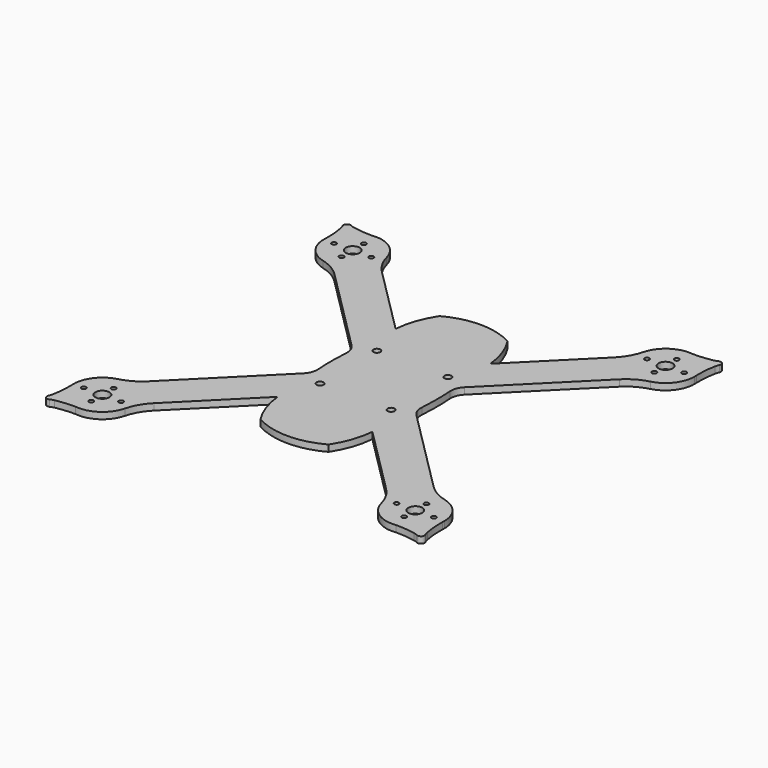
from build123d import *

# Parameters (mm, degrees)
F0_R     = 1
F0_R_2   = 3
F0_R_3   = 1.5
F1_DEPTH = 2.8


# Not quite as in the source:
# - a feature names something its author has since deleted; it is built from what else it names


with BuildPart() as f1:
    # F0 (on Top) → F1 (new body)
    with BuildSketch(Plane.XY):
        with BuildLine():
            ThreePointArc((-24.2769210382, 12.9632125392), (-22.6715914724, 10.4692673994), (-22.2430782145, 7.5344383136))
            add(Edge.make_bspline(
                [(-22.2430782145, 7.5344383136), (-22.7598893965, 0), (-22.2430782145, -7.5344383136)],
                knots=[1.419531369, 1.419531369, 1.419531369, 1.7220612846, 1.7220612846, 1.7220612846], degree=2, weights=[1, 0.988581254, 1]))
            ThreePointArc((-22.2430782145, -7.5344383136), (-22.6715914724, -10.4692673994), (-24.2769210382, -12.9632125392))
            Line((-24.2769210382, -12.9632125392), (-61.1647365726, -49.8510280737))
            ThreePointArc((-61.1647365726, -49.8510280737), (-65.3840934292, -53.0737552924), (-70.3027318987, -55.0727396886))
            ThreePointArc((-70.3027318987, -55.0727396886), (-77.058080165, -59.5215452578), (-79.6751442127, -67.1751442127))
            ThreePointArc((-79.6751442127, -67.1751442127), (-79.6503390116, -67.6938343507), (-79.6320011275, -68.2127933849))
            ThreePointArc((-79.6320011275, -68.2127933849), (-79.7454623748, -72.7266284611), (-80.3467756366, -77.2016706856))
            ThreePointArc((-80.3467756366, -77.2016706856), (-80.5705641186, -78.0710076077), (-80.9037667053, -78.9045566495))
            ThreePointArc((-80.9037667053, -78.9045566495), (-80.607151465, -80.6131466395), (-78.8969122154, -80.9000997088))
            ThreePointArc((-78.8969122154, -80.9000997088), (-78.065259844, -80.5621909904), (-77.1972017245, -80.3334923456))
            ThreePointArc((-77.1972017245, -80.3334923456), (-73.0608106601, -79.7368187673), (-68.8854512989, -79.5575853965))
            ThreePointArc((-68.8854512989, -79.5575853965), (-60.2172709309, -77.5596518753), (-55.0727396886, -70.3027318987))
            ThreePointArc((-55.0727396886, -70.3027318987), (-53.0737552924, -65.3840934292), (-49.8510280737, -61.1647365726))
            Line((-49.8510280737, -61.1647365726), (-20.3225413072, -31.6362498062))
            ThreePointArc((-20.3225413072, -31.6362498062), (-18.4728822052, -40.1836633503), (-14.6194240078, -48.0341650546))
            ThreePointArc((-14.6194240078, -48.0341650546), (0, -51.7838309168), (14.6194240078, -48.0341650546))
            ThreePointArc((14.6194240078, -48.0341650546), (18.4728822052, -40.1836633503), (20.3225413072, -31.6362498062))
            Line((20.3225413072, -31.6362498062), (49.8510280737, -61.1647365726))
            ThreePointArc((49.8510280737, -61.1647365726), (53.0737552924, -65.3840934292), (55.0727396886, -70.3027318987))
            ThreePointArc((55.0727396886, -70.3027318987), (60.2172709309, -77.5596518753), (68.8854512989, -79.5575853965))
            ThreePointArc((68.8854512989, -79.5575853965), (73.0608106601, -79.7368187673), (77.1972017245, -80.3334923456))
            ThreePointArc((77.1972017245, -80.3334923456), (78.065259844, -80.5621909904), (78.8969122154, -80.9000997088))
            ThreePointArc((78.8969122154, -80.9000997088), (80.607151465, -80.6131466395), (80.9037667053, -78.9045566495))
            ThreePointArc((80.9037667053, -78.9045566495), (80.5705641186, -78.0710076077), (80.3467756366, -77.2016706856))
            ThreePointArc((80.3467756366, -77.2016706856), (79.7454623748, -72.7266284611), (79.6320011275, -68.2127933849))
            ThreePointArc((79.6320011275, -68.2127933849), (79.6503390116, -67.6938343507), (79.6751442127, -67.1751442127))
            ThreePointArc((79.6751442127, -67.1751442127), (77.058080165, -59.5215452578), (70.3027318987, -55.0727396886))
            ThreePointArc((70.3027318987, -55.0727396886), (65.3840934292, -53.0737552924), (61.1647365726, -49.8510280737))
            Line((61.1647365726, -49.8510280737), (24.2769210382, -12.9632125392))
            ThreePointArc((24.2769210382, -12.9632125392), (22.6715914724, -10.4692673994), (22.2430782145, -7.5344383136))
            add(Edge.make_bspline(
                [(22.2430782145, -7.5344383136), (22.7598893965, 0), (22.2430782145, 7.5344383136)],
                knots=[4.5611240226, 4.5611240226, 4.5611240226, 4.8636539382, 4.8636539382, 4.8636539382], degree=2, weights=[1, 0.988581254, 1]))
            ThreePointArc((22.2430782145, 7.5344383136), (22.6715914724, 10.4692673994), (24.2769210382, 12.9632125392))
            Line((24.2769210382, 12.9632125392), (61.1647365726, 49.8510280737))
            ThreePointArc((61.1647365726, 49.8510280737), (65.3840934292, 53.0737552924), (70.3027318987, 55.0727396886))
            ThreePointArc((70.3027318987, 55.0727396886), (77.058080165, 59.5215452578), (79.6751442127, 67.1751442127))
            ThreePointArc((79.6751442127, 67.1751442127), (79.6503390116, 67.6938343507), (79.6320011275, 68.2127933849))
            ThreePointArc((79.6320011275, 68.2127933849), (79.7454623748, 72.7266284611), (80.3467756366, 77.2016706856))
            ThreePointArc((80.3467756366, 77.2016706856), (80.5705641186, 78.0710076077), (80.9037667053, 78.9045566495))
            ThreePointArc((80.9037667053, 78.9045566495), (80.607151465, 80.6131466395), (78.8969122154, 80.9000997088))
            ThreePointArc((78.8969122154, 80.9000997088), (78.065259844, 80.5621909904), (77.1972017245, 80.3334923456))
            ThreePointArc((77.1972017245, 80.3334923456), (73.0608106601, 79.7368187673), (68.8854512989, 79.5575853965))
            ThreePointArc((68.8854512989, 79.5575853965), (60.2172709309, 77.5596518753), (55.0727396886, 70.3027318987))
            ThreePointArc((55.0727396886, 70.3027318987), (53.0737552924, 65.3840934292), (49.8510280737, 61.1647365726))
            Line((49.8510280737, 61.1647365726), (20.3225413072, 31.6362498062))
            ThreePointArc((20.3225413072, 31.6362498062), (18.4728822052, 40.1836633503), (14.6194240078, 48.0341650546))
            ThreePointArc((14.6194240078, 48.0341650546), (0, 51.7838309168), (-14.6194240078, 48.0341650546))
            ThreePointArc((-14.6194240078, 48.0341650546), (-18.4728822052, 40.1836633503), (-20.3225413072, 31.6362498062))
            Line((-20.3225413072, 31.6362498062), (-49.8510280737, 61.1647365726))
            ThreePointArc((-49.8510280737, 61.1647365726), (-53.0737552924, 65.3840934292), (-55.0727396886, 70.3027318987))
            ThreePointArc((-55.0727396886, 70.3027318987), (-60.2172709309, 77.5596518753), (-68.8854512989, 79.5575853965))
            ThreePointArc((-68.8854512989, 79.5575853965), (-73.0608106601, 79.7368187673), (-77.1972017245, 80.3334923456))
            ThreePointArc((-77.1972017245, 80.3334923456), (-78.065259844, 80.5621909904), (-78.8969122154, 80.9000997088))
            ThreePointArc((-78.8969122154, 80.9000997088), (-80.607151465, 80.6131466395), (-80.9037667053, 78.9045566495))
            ThreePointArc((-80.9037667053, 78.9045566495), (-80.5705641186, 78.0710076077), (-80.3467756366, 77.2016706856))
            ThreePointArc((-80.3467756366, 77.2016706856), (-79.7454623748, 72.7266284611), (-79.6320011275, 68.2127933849))
            ThreePointArc((-79.6320011275, 68.2127933849), (-79.6503390116, 67.6938343507), (-79.6751442127, 67.1751442127))
            ThreePointArc((-79.6751442127, 67.1751442127), (-77.058080165, 59.5215452578), (-70.3027318987, 55.0727396886))
            ThreePointArc((-70.3027318987, 55.0727396886), (-65.3840934292, 53.0737552924), (-61.1647365726, 49.8510280737))
            Line((-61.1647365726, 49.8510280737), (-24.2769210382, 12.9632125392))
        make_face()
        with Locations((-67.1751442127, -73.1751442127)):
            Circle(F0_R, mode=Mode.SUBTRACT)
        with Locations((-75.1751442127, -67.1751442127)):
            Circle(F0_R, mode=Mode.SUBTRACT)
        with Locations((-67.1751442127, -67.1751442127)):
            Circle(F0_R_2, mode=Mode.SUBTRACT)
        with Locations((-67.1751442127, -61.1751442127)):
            Circle(F0_R, mode=Mode.SUBTRACT)
        with Locations((-59.1751442127, -67.1751442127)):
            Circle(F0_R, mode=Mode.SUBTRACT)
        with Locations((-15.25, -15.25)):
            Circle(F0_R_3, mode=Mode.SUBTRACT)
        with Locations((59.1751442127, -67.1751442127)):
            Circle(F0_R, mode=Mode.SUBTRACT)
        with Locations((67.1751442127, -73.1751442127)):
            Circle(F0_R, mode=Mode.SUBTRACT)
        with Locations((67.1751442127, -67.1751442127)):
            Circle(F0_R_2, mode=Mode.SUBTRACT)
        with Locations((67.1751442127, -61.1751442127)):
            Circle(F0_R, mode=Mode.SUBTRACT)
        with Locations((75.1751442127, -67.1751442127)):
            Circle(F0_R, mode=Mode.SUBTRACT)
        with Locations((15.25, -15.25)):
            Circle(F0_R_3, mode=Mode.SUBTRACT)
        with Locations((-15.25, 15.25)):
            Circle(F0_R_3, mode=Mode.SUBTRACT)
        with Locations((-75.1751442127, 67.1751442127)):
            Circle(F0_R, mode=Mode.SUBTRACT)
        with Locations((-67.1751442127, 61.1751442127)):
            Circle(F0_R, mode=Mode.SUBTRACT)
        with Locations((-67.1751442127, 67.1751442127)):
            Circle(F0_R_2, mode=Mode.SUBTRACT)
        with Locations((-67.1751442127, 73.1751442127)):
            Circle(F0_R, mode=Mode.SUBTRACT)
        with Locations((-59.1751442127, 67.1751442127)):
            Circle(F0_R, mode=Mode.SUBTRACT)
        with Locations((15.25, 15.25)):
            Circle(F0_R_3, mode=Mode.SUBTRACT)
        with Locations((59.1751442127, 67.1751442127)):
            Circle(F0_R, mode=Mode.SUBTRACT)
        with Locations((67.1751442127, 61.1751442127)):
            Circle(F0_R, mode=Mode.SUBTRACT)
        with Locations((67.1751442127, 67.1751442127)):
            Circle(F0_R_2, mode=Mode.SUBTRACT)
        with Locations((75.1751442127, 67.1751442127)):
            Circle(F0_R, mode=Mode.SUBTRACT)
        with Locations((67.1751442127, 73.1751442127)):
            Circle(F0_R, mode=Mode.SUBTRACT)
    extrude(amount=F1_DEPTH)


solid = f1.part
